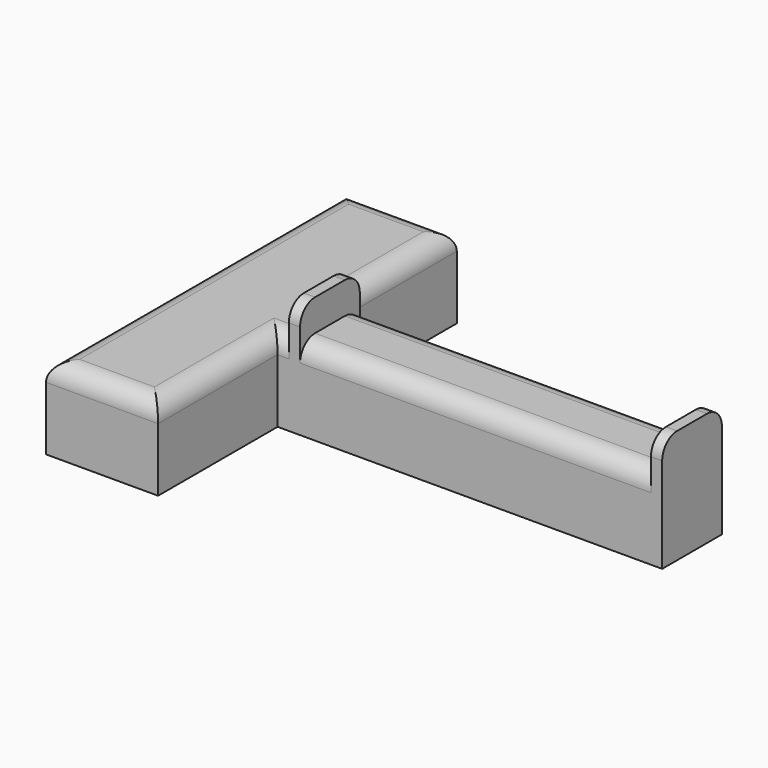
from build123d import *

# Parameters (mm, degrees)
F0_R     = 6.25
F0_W     = 15
F0_H     = 20
F0_W_2   = 93.98
F0_W_3   = 3.02
F0_W_4   = 3
F1_DEPTH = 22
F2_DEPTH = 30.48
F3_DEPTH = 18
F4_SIZE  = 4
F5_R     = 5


with BuildPart() as f1:
    # F0 (on Top) → F1 (new body)
    with BuildSketch(Plane.XY):
        Polygon((15, 10), (15, 50), (-15, 50), (-15, -50), (15, -50), (15, -10), (0, -10), (0, 10), align=None)
        with Locations((0, -35)):
            Circle(F0_R, mode=Mode.SUBTRACT)
        with Locations((0, 35)):
            Circle(F0_R, mode=Mode.SUBTRACT)
        with Locations((7.5, 0)):
            Rectangle(F0_W, F0_H)
        with Locations((68.01, 0)):
            Rectangle(F0_W_2, F0_H)
        with Locations((0, -35)):
            Circle(F0_R)
        with Locations((0, 35)):
            Circle(F0_R)
        with Locations((16.51, 0)):
            Rectangle(F0_W_3, F0_H)
        with Locations((19.52, 0)):
            Rectangle(F0_W_4, F0_H)
    extrude(amount=F1_DEPTH)

    # F0 (on Top) → F2 (join)
    with BuildSketch(Plane.XY):
        with Locations((116.5, 0)):
            Rectangle(F0_W_4, F0_H)
        with Locations((19.52, 0)):
            Rectangle(F0_W_4, F0_H)
    extrude(amount=F2_DEPTH)

    # F0 (on Top) → F3 (cut)
    with BuildSketch(Plane.XY):
        with Locations((0, -35)):
            Circle(F0_R)
        with Locations((0, 35)):
            Circle(F0_R)
    extrude(amount=F3_DEPTH, mode=Mode.SUBTRACT)

    # F4
    f4_edges = [f1.edges().sort_by_distance(p)[0] for p in [
        (-6.25, -35, 18),
        (-6.25, 35, 18),
    ]]
    chamfer(f4_edges, length=F4_SIZE)

    # F5
    f5_edges = [f1.edges().sort_by_distance(p)[0] for p in [
        (68.01, -10, 22),
        (68.01, 10, 22),
        (116.5, -10, 30.48),
        (116.5, 10, 30.48),
        (15, -30, 22),
        (15, 30, 22),
        (-15, 0, 22),
        (0, -50, 22),
        (0, 50, 22),
        (19.52, -10, 30.48),
        (19.52, 10, 30.48),
        (16.51, 10, 22),
        (16.51, -10, 22),
    ]]
    fillet(f5_edges, radius=F5_R)


solid = f1.part
